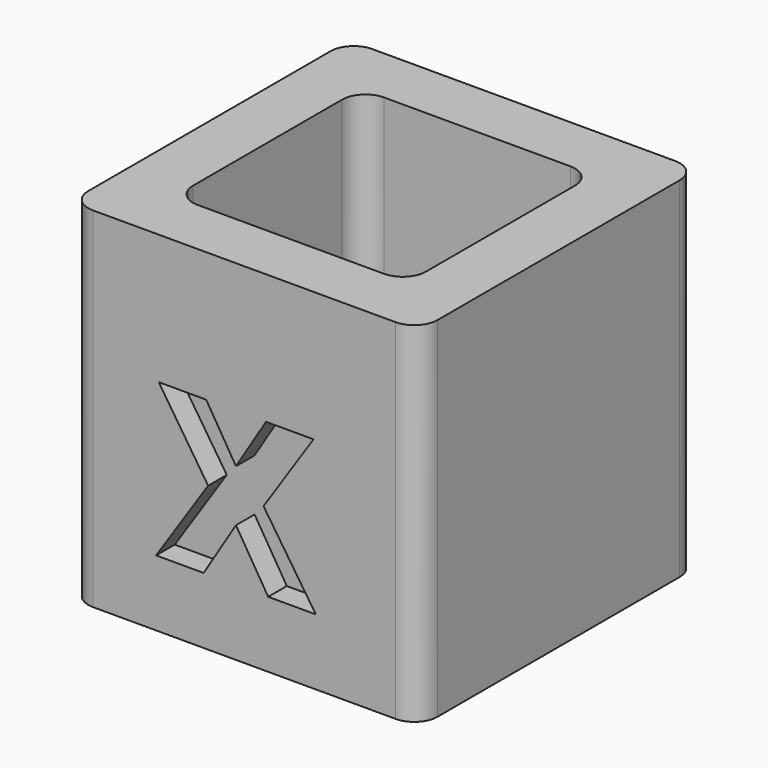
from build123d import *

# Parameters (mm, degrees)
F0_W         = 15
F0_H         = 15
F0_W_2       = 10
F0_H_2       = 10
F1_DEPTH     = 15
F2_R         = 1
F4_TEXT_SIZE = 9.9445400167
F5_DEPTH     = 1
F3_TEXT_SIZE = 12.0653984292
F6_DEPTH     = 1


# Not quite as in the source:
# - Text() gives the source's letters only with a copy of the font that has no kerning and outlines rounded to 1/6400 em; it was checked with that copy


with BuildPart() as f1:
    # F0 (on Top) → F1 (new body)
    with BuildSketch(Plane.XY):
        Rectangle(F0_W, F0_H)
        Rectangle(F0_W_2, F0_H_2, mode=Mode.SUBTRACT)
    extrude(amount=F1_DEPTH)

    # F2
    f2_edges = [f1.edges().sort_by_distance(p)[0] for p in [
        (-7.5, 7.5, 7.5),
        (-7.5, -7.5, 7.5),
        (7.5, -7.5, 7.5),
        (7.5, 7.5, 7.5),
        (5, 5, 7.5),
        (-5, 5, 7.5),
        (5, -5, 7.5),
        (-5, -5, 7.5),
    ]]
    fillet(f2_edges, radius=F2_R)

    # F4 (on face) → F5 (cut)
    with BuildSketch(Plane(origin=(-7.5, 0, 0), x_dir=(0, -1, 0), z_dir=(-1, 0, 0))):
        with Locations((-3.1511761178, 4.2843950179)):
            Text('y', F4_TEXT_SIZE, font='Open Sans', font_style=FontStyle.BOLD, text_align=(TextAlign.LEFT, TextAlign.BOTTOM))
    extrude(amount=-F5_DEPTH, mode=Mode.SUBTRACT)

    # F3 (on face) → F6 (cut)
    with BuildSketch(Plane.XZ.offset(7.5)):
        with Locations((-3.8453135639, 2.8370781802)):
            Text('x', F3_TEXT_SIZE, font='Open Sans', font_style=FontStyle.BOLD, text_align=(TextAlign.LEFT, TextAlign.BOTTOM))
    extrude(amount=-F6_DEPTH, mode=Mode.SUBTRACT)


solid = f1.part
